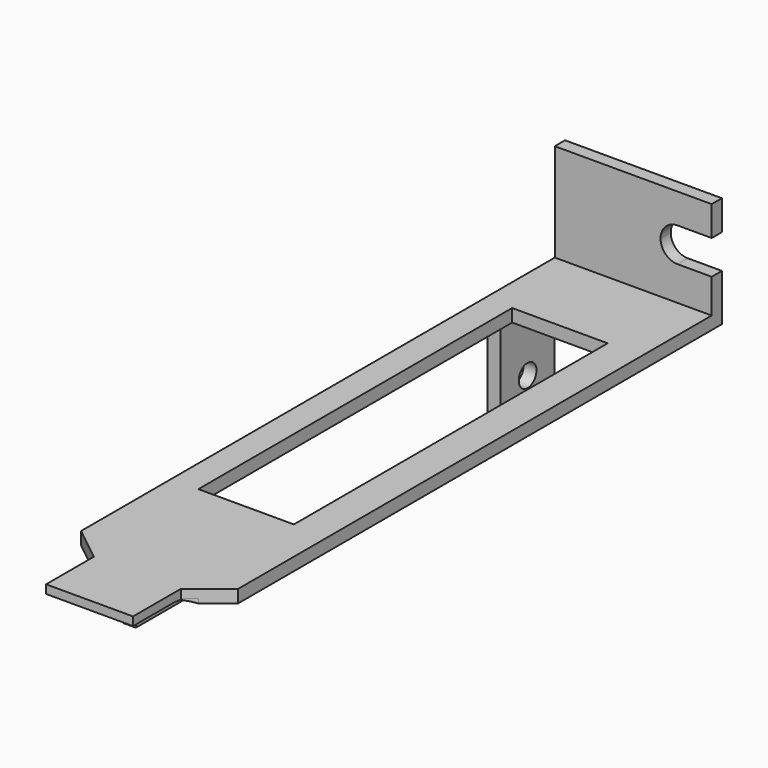
from build123d import *

# Parameters (mm, degrees)
F0_W          = 10.2
F0_H          = 7
F1_DEPTH      = 1.5
F2_W          = 11.2
F2_H          = 46
F3_DEPTH      = 25
F4_W          = 1.5
F4_H          = 70.9369339572
F5_DEPTH      = 10.5
F6_W          = 45.52
F6_H          = 10.5
F6_R          = 1.3
F6_W_2        = 3.43
F6_W_3        = 6.1469339572
F7_DEPTH      = 25
F9_DEPTH      = 0.5
F10_T4_DEPTH  = 23.6102213202
F10_T10_DEPTH = 23.6102213202
F11_W         = 18.4
F11_H         = 1.5
F12_DEPTH     = 11.5
F14_DEPTH     = 1.5


# Not quite as in the source:
# - a fillet or chamfer that OpenCascade refuses, or shapes differently, is made with other operations: its cross-section is extruded or revolved along the edge and cut away or added


with BuildPart() as f1:
    # F0 (on Top) → F1 (new body)
    with BuildSketch(Plane.XY):
        Polygon((12.9583973216, 44.6379526287), (-5.4416026784, 44.6379526287), (-5.4416026784, -26.2989813285), (-1.3416026784, -29.5620473713), (8.8583973216, -29.5620473713), (12.9583973216, -26.2989813285), align=None)
        with Locations((3.7583973216, -33.0620473713)):
            Rectangle(F0_W, F0_H)
    extrude(amount=F1_DEPTH)

    # F2 (on face) → F3 (cut)
    with BuildSketch(Plane.XY.offset(1.5)):
        with Locations((3.3583973216, 9.8879526287)):
            Rectangle(F2_W, F2_H)
    extrude(amount=-F3_DEPTH, mode=Mode.SUBTRACT)

    # F4 (on face) → F5 (join)
    with BuildSketch(Plane(origin=(0, 0, 0), x_dir=(1, 0, 0), z_dir=(0, 0, -1))):
        with Locations((-4.6916026784, -9.1694856501)):
            Rectangle(F4_W, F4_H)
    extrude(amount=F5_DEPTH)

    # F6 (on face) → F7 (cut)
    with BuildSketch(Plane.YZ.offset(-3.9416026784)):
        with Locations((10.5479526287, -5.25)):
            Rectangle(F6_W, F6_H)
        with Locations((-16.1820473713, -7.8)):
            Circle(F6_R)
        with Locations((37.2779526287, -7.8)):
            Circle(F6_R)
        with Locations((42.9229526287, -5.25)):
            Rectangle(F6_W_2, F6_H)
        with Locations((-23.2255143499, -5.25)):
            Rectangle(F6_W_3, F6_H)
    extrude(amount=-F7_DEPTH, mode=Mode.SUBTRACT)

    # F8 (on face) → F9 (cut)
    with BuildSketch(Plane(origin=(0, 0, 0), x_dir=(1, 0, 0), z_dir=(0, 0, -1))):
        Polygon((-1.3416026784, 29.5620473713), (-2.5980896591, 28.5620473713), (10.1148843023, 28.5620473713), (8.8583973216, 29.5620473713), (8.8583973216, 36.5620473713), (-1.3416026784, 36.5620473713), align=None)
    extrude(amount=-F9_DEPTH, mode=Mode.SUBTRACT)

    # F10: fillet of radius 5 on 1 edges, made by hand


with BuildPart() as f10_tool2:
    # F10_s3 → F10_t4 (new body)
    with BuildSketch(Plane.YZ.offset(-8.0467133385)):
        with BuildLine():
            ThreePointArc((-30.7414968431, 0.5), (-29.6234628544, 0.3733971724), (-28.5620473713, 0))
            Line((-28.5620473713, 0), (-28.5620473713, 0.5))
            Line((-28.5620473713, 0.5), (-30.7414968431, 0.5))
        make_face()
    extrude(amount=F10_T4_DEPTH)

    split(bisect_by=Plane.YZ.offset(8.8583973216), keep=Keep.BOTTOM)

    split(bisect_by=Plane(origin=(-14.9242028331, -18.7520665571, 0), x_dir=(0, 0, 1), z_dir=(0.6227225273, 0.7824427481, 0)), keep=Keep.TOP)


with BuildPart() as f1_1:
    add(f1.part)

    # F10_t1: union F10_tool2
    add(f10_tool2.part)


with BuildPart() as f10_tool8:
    # F10_s9 → F10_t10 (new body)
    with BuildSketch(Plane.YZ.offset(-8.0467133385)):
        with BuildLine():
            ThreePointArc((-30.7414968431, 0.5), (-29.6234628544, 0.3733971724), (-28.5620473713, 0))
            Line((-28.5620473713, 0), (-28.5620473713, 0.5))
            Line((-28.5620473713, 0.5), (-30.7414968431, 0.5))
        make_face()
    extrude(amount=F10_T10_DEPTH)

    split(bisect_by=Plane(origin=(17.8390906107, -22.4145850999, 0), x_dir=(0, 0, 1), z_dir=(-0.6227225273, 0.7824427481, 0)), keep=Keep.TOP)

    split(bisect_by=Plane.YZ.offset(-1.3416026784), keep=Keep.TOP)


with BuildPart() as f1_2:
    add(f1_1.part)

    # F10_t7: union F10_tool8
    add(f10_tool8.part)

    # F11 (on face) → F12 (join)
    with BuildSketch(Plane.XY.offset(1.5)):
        with Locations((3.7583973216, 43.8879526287)):
            Rectangle(F11_W, F11_H)
    extrude(amount=F12_DEPTH)

    # F13 (on face) → F14 (cut, through all)
    with BuildSketch(Plane(origin=(0, 44.6379526287, 0), x_dir=(-1, 0, 0), z_dir=(0, 1, 0))):
        with BuildLine():
            ThreePointArc((-6.9583973216, 7.5), (-7.5441837593, 8.9142135624), (-8.9583973216, 9.5))
            ThreePointArc((-8.9583973216, 9.5), (-10.9583973216, 7.5), (-8.9583973216, 5.5))
            ThreePointArc((-8.9583973216, 5.5), (-7.5441837593, 6.0857864376), (-6.9583973216, 7.5))
        make_face()
        with BuildLine():
            Line((-8.9583973216, 9.5), (-12.9583973216, 9.5))
            Line((-12.9583973216, 9.5), (-12.9583973216, 5.5))
            Line((-12.9583973216, 5.5), (-8.9583973216, 5.5))
            ThreePointArc((-8.9583973216, 5.5), (-10.9583973216, 7.5), (-8.9583973216, 9.5))
        make_face()
    extrude(amount=-F14_DEPTH, mode=Mode.SUBTRACT)


solid = f1_2.part
